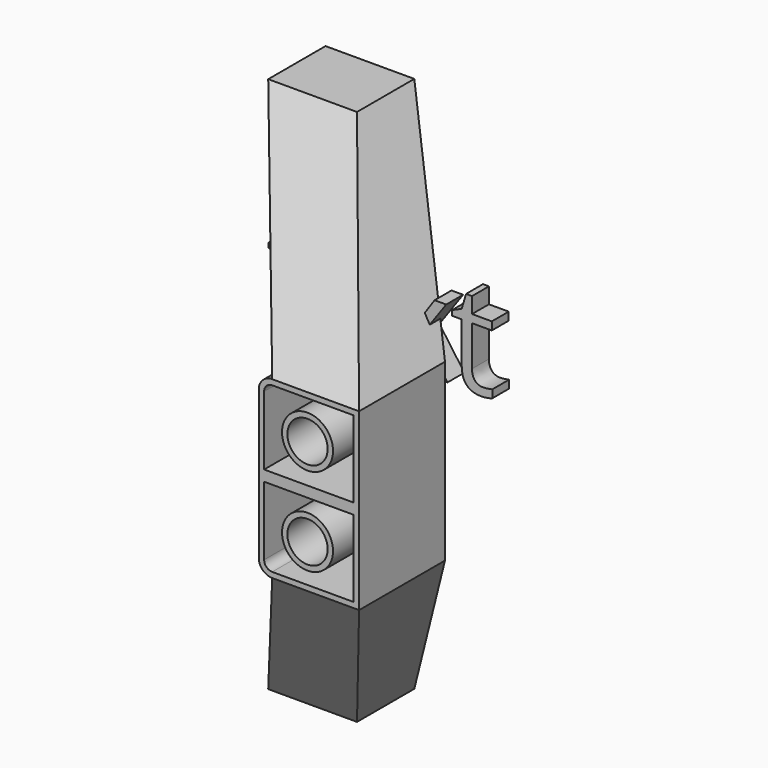
from build123d import *

# Parameters (mm, degrees)
F0_R         = 9.5240178451
F1_DEPTH     = 50.8
F4_T         = -2.54
F3_W         = 41.998770088
F3_H         = 33.8853425346
F1_FACE_W    = 41.0989107728
F1_FACE_H    = 50.8
F7_TEXT_SIZE = 60.2810436653
F8_DEPTH     = 10


# Not quite as in the source:
# - Text() gives the source's letters only with a copy of the font that has no kerning and outlines rounded to 1/6400 em; it was checked with that copy


with BuildPart() as f1:
    # F0 (on Front) → F1 (new body)
    with BuildSketch(Plane.XZ):
        with BuildLine():
            Line((0, 35.0477280259), (0, 0))
            Line((0, 0), (47.4489107728, 0))
            Line((47.4489107728, 0), (47.4489107728, 41.3977280259))
            Line((47.4489107728, 41.3977280259), (6.35, 41.3977280259))
            ThreePointArc((6.35, 41.3977280259), (1.8598719395, 39.5378560864), (0, 35.0477280259))
        make_face()
        with Locations((23.0521019548, 20.8429433405)):
            Circle(F0_R, mode=Mode.SUBTRACT)
    extrude(amount=F1_DEPTH)

    # F4
    f4_openings = [f1.faces().sort_by_distance(p)[0] for p in [
        (0.629696, -50.8, 17.523864),
    ]]
    offset(amount=F4_T, openings=f4_openings)

    # F3 (on offset) → F5 section 0
    with BuildSketch(Plane.XY.offset(127)):
        with Locations((-20.999385044, 24.2247369606)):
            Rectangle(F3_W, F3_H)
    # F1_face (on face) → F5 section 1
    with BuildSketch(Plane(origin=(26.8994553864, -25.4, 41.3977280259), x_dir=(1, 0, 0), z_dir=(0, 0, 1))):
        Rectangle(F1_FACE_W, F1_FACE_H)
    loft()

    # F6: F1 across plane


with BuildPart() as f1_1:
    add(f1.part)
    add(f1.part.mirror(Plane.XY))

    # F7 (on Front) → F8 (join)
    with BuildSketch(Plane.XZ):
        with Locations((-36.8685126305, 33.1316143274)):
            Text('text', F7_TEXT_SIZE, font='Open Sans', text_align=(TextAlign.LEFT, TextAlign.BOTTOM))
    extrude(amount=-F8_DEPTH)


solid = f1_1.part
